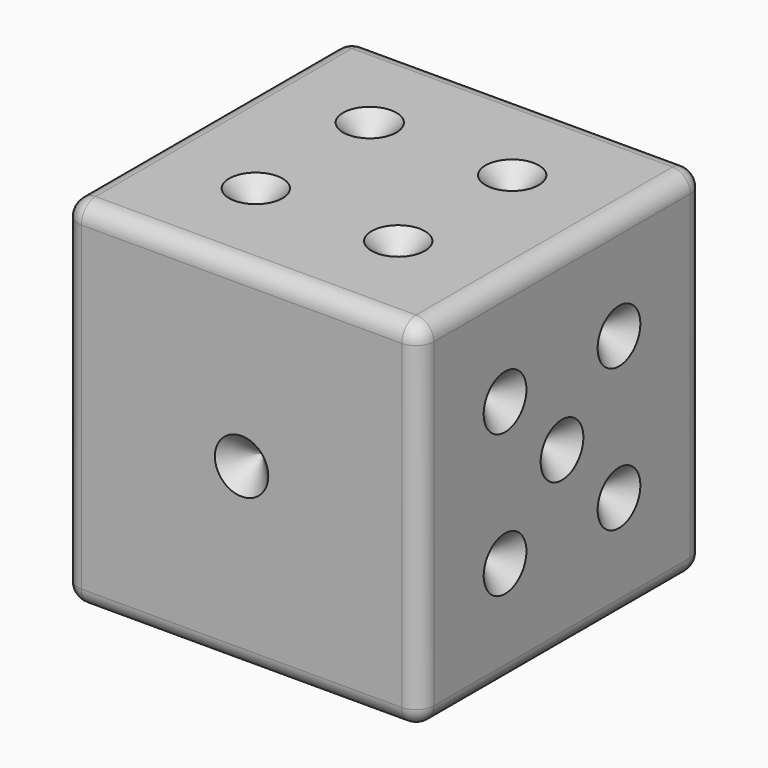
from build123d import *

# Parameters (mm, degrees)
F0_W      = 20
F0_H      = 20
F1_DEPTH  = 20
F2_R      = 1.5
F3_DEPTH  = 1.5
F4_R      = 1.5
F5_DEPTH  = 1.5
F6_R      = 1.5
F7_DEPTH  = 1.5
F8_R      = 1.5
F9_DEPTH  = 1.5
F10_R     = 1.5
F11_DEPTH = 1.5
F12_R     = 1.5
F13_DEPTH = 1.5
F14_R     = 1
F15_SIZE  = 1.49999


# Not quite as in the source:
# - a fillet or chamfer is up to 0.001 mm smaller than in the source, because OpenCascade refuses the exact size


with BuildPart() as f1:
    # F0 (on Top) → F1 (new body)
    with BuildSketch(Plane.XY):
        with Locations((10, 10)):
            Rectangle(F0_W, F0_H)
    extrude(amount=F1_DEPTH)

    # F2 (on face) → F3 (cut)
    with BuildSketch(Plane.XZ):
        with Locations((10, 10)):
            Circle(F2_R)
    extrude(amount=-F3_DEPTH, mode=Mode.SUBTRACT)

    # F4 (on face) → F5 (cut)
    with BuildSketch(Plane.XY.offset(20)):
        with Locations((6, 14)):
            Circle(F4_R)
        with Locations((6, 6)):
            Circle(F4_R)
        with Locations((14, 6)):
            Circle(F4_R)
        with Locations((14, 14)):
            Circle(F4_R)
    extrude(amount=-F5_DEPTH, mode=Mode.SUBTRACT)

    # F6 (on face) → F7 (cut)
    with BuildSketch(Plane.YZ.offset(20)):
        with Locations((6, 14)):
            Circle(F6_R)
        with Locations((6, 6)):
            Circle(F6_R)
        with Locations((14, 6)):
            Circle(F6_R)
        with Locations((14, 14)):
            Circle(F6_R)
        with Locations((10, 10)):
            Circle(F6_R)
    extrude(amount=-F7_DEPTH, mode=Mode.SUBTRACT)

    # F8 (on face) → F9 (cut)
    with BuildSketch(Plane(origin=(0, 20, 0), x_dir=(-1, 0, 0), z_dir=(0, 1, 0))):
        with Locations((-14, 14)):
            Circle(F8_R)
        with Locations((-14, 6)):
            Circle(F8_R)
        with Locations((-14, 10)):
            Circle(F8_R)
        with Locations((-6, 14)):
            Circle(F8_R)
        with Locations((-6, 10)):
            Circle(F8_R)
        with Locations((-6, 6)):
            Circle(F8_R)
    extrude(amount=-F9_DEPTH, mode=Mode.SUBTRACT)

    # F10 (on face) → F11 (cut)
    with BuildSketch(Plane(origin=(0, 0, 0), x_dir=(0, -1, 0), z_dir=(-1, 0, 0))):
        with Locations((-14, 14)):
            Circle(F10_R)
        with Locations((-6, 6)):
            Circle(F10_R)
    extrude(amount=-F11_DEPTH, mode=Mode.SUBTRACT)

    # F12 (on face) → F13 (cut)
    with BuildSketch(Plane(origin=(0, 0, 0), x_dir=(1, 0, 0), z_dir=(0, 0, -1))):
        with Locations((6, -6)):
            Circle(F12_R)
        with Locations((14, -14)):
            Circle(F12_R)
        with Locations((10, -10)):
            Circle(F12_R)
    extrude(amount=-F13_DEPTH, mode=Mode.SUBTRACT)

    # F14
    f14_edges = [f1.edges().sort_by_distance(p)[0] for p in [
        (0, 10, 20),
        (20, 10, 20),
        (10, 0, 20),
        (10, 0, 0),
        (0, 10, 0),
        (10, 20, 0),
        (10, 20, 20),
        (20, 20, 10),
        (0, 20, 10),
        (20, 0, 10),
        (0, 0, 10),
        (20, 10, 0),
    ]]
    fillet(f14_edges, radius=F14_R)

    # F15 (size 1.5 in the source; OpenCascade refuses exactly that, so slightly less here)
    f15_edges = [f1.edges().sort_by_distance(p)[0] for p in [
        (8.5, 1.5, 10),
        (4.5, 14, 18.5),
        (4.5, 6, 18.5),
        (12.5, 6, 18.5),
        (12.5, 14, 18.5),
        (18.5, 4.5, 6),
        (18.5, 4.5, 14),
        (18.5, 12.5, 14),
        (18.5, 12.5, 6),
        (18.5, 8.5, 10),
        (15.5, 18.5, 14),
        (15.5, 18.5, 10),
        (15.5, 18.5, 6),
        (7.5, 18.5, 6),
        (7.5, 18.5, 10),
        (7.5, 18.5, 14),
        (1.5, 15.5, 14),
        (1.5, 7.5, 6),
        (4.5, 6, 1.5),
        (8.5, 10, 1.5),
        (12.5, 14, 1.5),
    ]]
    chamfer(f15_edges, length=F15_SIZE)


solid = f1.part
